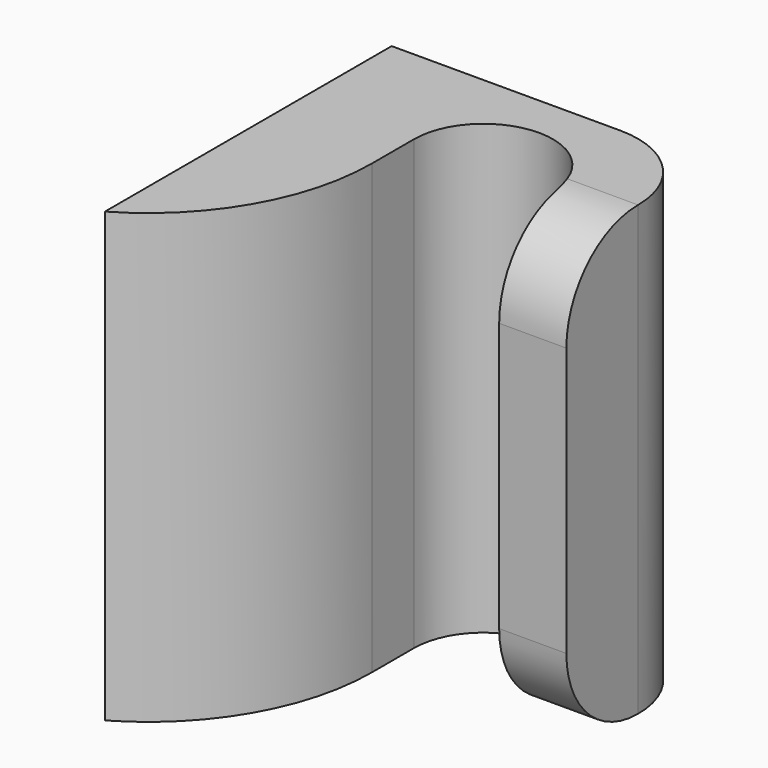
from build123d import *

# Parameters (mm, degrees)
F1_DEPTH    = 12.7
F2_R        = 2.54
F3_T1_DEPTH = 40.1963065702
F4_R        = 2.54


# Not quite as in the source:
# - a fillet or chamfer that OpenCascade refuses, or shapes differently, is made with other operations: its cross-section is extruded or revolved along the edge and cut away or added


with BuildPart() as f1:
    # F0 (on Top) → F1 (new body)
    with BuildSketch(Plane.XY):
        with BuildLine():
            Line((0, 5.08), (0, -5.08))
            Line((0, -5.08), (3.175, -5.08))
            Line((3.175, -5.08), (3.175, 1.905))
            ThreePointArc((3.175, 1.905), (5.1435, 3.8735), (7.112, 1.905))
            Line((7.112, 1.905), (7.112, 0))
            Line((7.112, 0), (9.017, 0))
            Line((9.017, 0), (9.017, 5.08))
            Line((9.017, 5.08), (0, 5.08))
        make_face()
    extrude(amount=F1_DEPTH)

    # F2
    f2_edges = [f1.edges().sort_by_distance(p)[0] for p in [
        (9.017, 5.08, 6.35),
    ]]
    fillet(f2_edges, radius=F2_R)

    # F3: fillet of radius 6.35 on 1 edges, made by hand

    # F3_s2 → F3_t1 (cut)
    with BuildSketch(Plane.XY.offset(-13.7481532851)):
        with BuildLine():
            ThreePointArc((0, -5.08), (2.324261314, -2.755738686), (3.175, 0.419261314))
            Line((3.175, 0.419261314), (3.175, -5.08))
            Line((3.175, -5.08), (0, -5.08))
        make_face()
    extrude(amount=F3_T1_DEPTH, mode=Mode.SUBTRACT)

    # F4
    f4_edges = [f1.edges().sort_by_distance(p)[0] for p in [
        (8.0645, 0, 12.7),
        (8.0645, 0, 0),
    ]]
    fillet(f4_edges, radius=F4_R)


solid = f1.part
